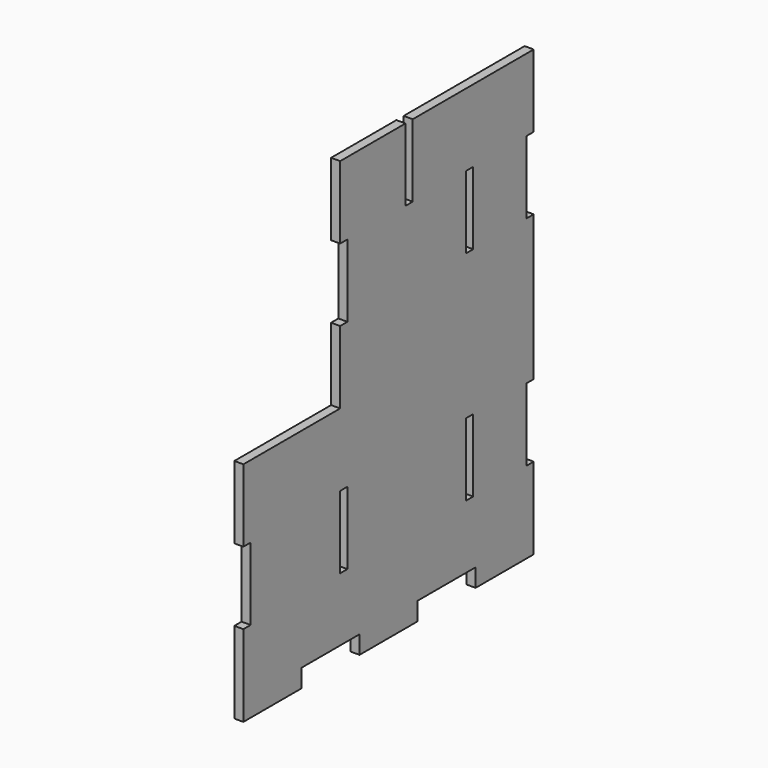
from build123d import *

# Parameters (mm, degrees)
F1_DEPTH = 19.05
F2_W     = 19.05
F2_H     = 152.4
F2_W_2   = 152.4
F2_H_2   = 38.1
F3_DEPTH = 19.05


# Not quite as in the source:
# - a length typed as a fraction of an inch, garbled in the dataset ("3 / 203.2 mm" for 3/8 in), is restored


with BuildPart() as f1:
    # F0 (on Right) → F1 (new body)
    with BuildSketch(Plane.YZ):
        Polygon((-127, 50.8), (-381, 50.8), (-381, -425.45), (381, -425.45), (381, 508), (-127, 508), align=None)
    extrude(amount=F1_DEPTH)

    # F2 (on face) → F3 (cut)
    with BuildSketch(Plane.YZ.offset(19.05)):
        with Locations((371.475, 279.4)):
            Rectangle(F2_W, F2_H)
        with Locations((371.475, -177.8)):
            Rectangle(F2_W, F2_H)
        with Locations((53.975, 431.8)):
            Rectangle(F2_W, F2_H)
        with Locations((-117.475, 279.4)):
            Rectangle(F2_W, F2_H)
        with Locations((212.725, 279.4)):
            Rectangle(F2_W, F2_H)
        with Locations((212.725, -177.8)):
            Rectangle(F2_W, F2_H)
        with Locations((-117.475, -177.8)):
            Rectangle(F2_W, F2_H)
        with Locations((-371.475, -177.8)):
            Rectangle(F2_W, F2_H)
        with Locations((152.4, -406.4)):
            Rectangle(F2_W_2, F2_H_2)
        with Locations((-152.4, -406.4)):
            Rectangle(F2_W_2, F2_H_2)
    extrude(amount=-F3_DEPTH, mode=Mode.SUBTRACT)


solid = f1.part
